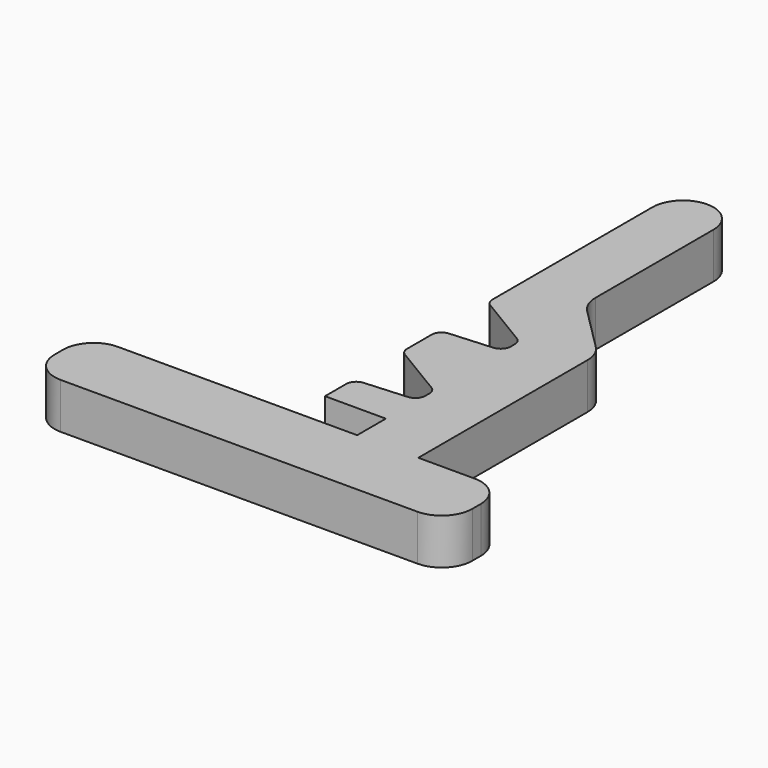
from build123d import *

# Parameters (mm, degrees)
F0_W     = 5.08
F0_H     = 15.875
F1_DEPTH = 3.81
F2_R     = 2.53999
F3_R     = 0.8382


# Not quite as in the source:
# - two fillets or chamfers of one size are made in one step
# - a fillet or chamfer is up to 0.001 mm smaller than in the source, because OpenCascade refuses the exact size
# - a feature names something its author has since deleted; it is built from what else it names


with BuildPart() as f1:
    # F0 (on Top) → F1 (new body)
    with BuildSketch(Plane.XY):
        Polygon((22.4666253753, 12.2923628866), (17.399, 11.938), (27.559, 11.938), (27.559, 24.638), (22.479, 29.718), (17.399, 29.718), (17.399, 25.908), (22.4666253753, 22.86306348), (22.4666253753, 21.1823628866), (17.399, 20.828), (17.399, 17.018), (22.4666253753, 13.97306348), align=None)
        Polygon((0, 5.969), (0, 0), (34.798, 0), (34.798, 5.969), (27.559, 5.969), (27.559, 11.938), (17.399, 11.938), (17.399, 8.9535), (22.4666253753, 8.9535), (22.4666253753, 5.969), align=None)
        with Locations((19.939, 37.6555)):
            Rectangle(F0_W, F0_H)
    extrude(amount=F1_DEPTH)

    # F2 (radius 2.54 in the source; OpenCascade refuses exactly that, so slightly less here)
    f2_edges = [f1.edges().sort_by_distance(p)[0] for p in [
        (0, 0, 1.905),
        (34.798, 0, 1.905),
        (17.399, 45.593, 1.905),
        (22.479, 45.593, 1.905),
        (0, 5.969, 1.905),
        (34.798, 5.969, 1.905),
        (27.559, 24.638, 1.905),
        (22.479, 29.718, 1.905),
    ]]
    fillet(f2_edges, radius=F2_R)

    # F3
    f3_edges = [f1.edges().sort_by_distance(p)[0] for p in [
        (22.466625, 21.182363, 1.905),
        (22.466625, 22.863063, 1.905),
        (22.466625, 12.292363, 1.905),
        (22.466625, 13.973063, 1.905),
        (17.399, 11.938, 1.905),
        (17.399, 17.018, 1.905),
        (17.399, 20.828, 1.905),
        (17.399, 25.908, 1.905),
    ]]
    fillet(f3_edges, radius=F3_R)


solid = f1.part
